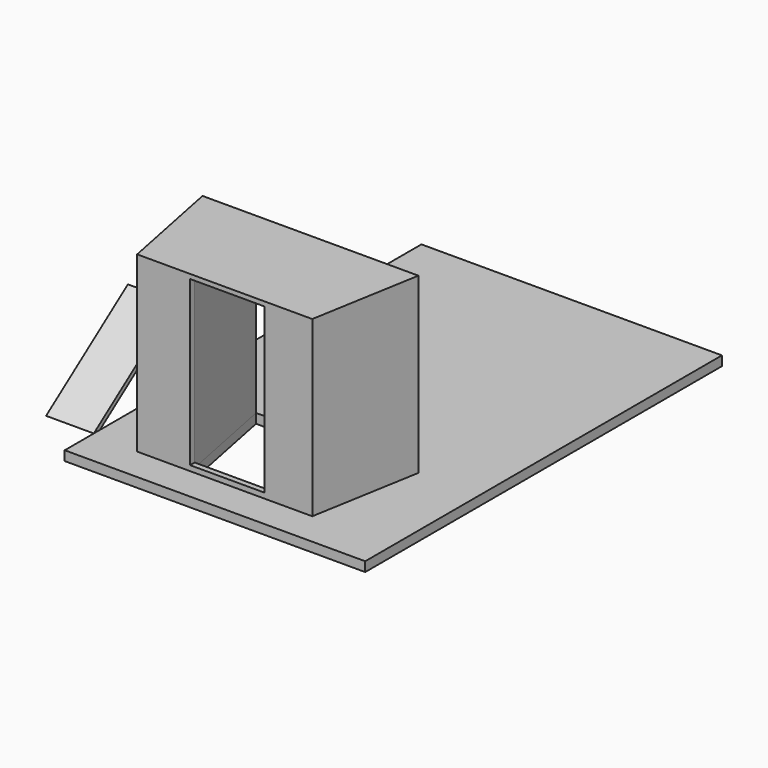
from build123d import *

# Parameters (mm, degrees)
F0_W        = 157.48
F0_H        = 233.68
F1_DEPTH    = 5
F3_DEPTH    = 91
F6_T        = 3
F6_T3_DEPTH = 64.2794708824
F6_T5_DEPTH = 72.7802281678
F6_T7_DEPTH = 63.9911646968
F4_W        = 61.3570176065
F4_H        = 85.9
F7_DEPTH    = 71
F8_DEPTH    = 27.4
F3_FACE1_W  = 58.2794708824
F3_FACE1_H  = 91
F3_FACE2_W  = 57.9911646968
F3_FACE2_H  = 91
F10_DEPTH   = 25


# Not quite as in the source:
# - a shell that OpenCascade refuses in one call is made with other operations: the cavity is built on its own and cut out


with BuildPart() as f1:
    # F0 (on Top) → F1 (new body)
    with BuildSketch(Plane.XY):
        with Locations((-51.8874652431, -0.1439023763)):
            Rectangle(F0_W, F0_H)
    extrude(amount=F1_DEPTH)

    # F2 (on face) → F3 (join)
    with BuildSketch(Plane.XY.offset(5)):
        Polygon((-93.2051390409, -42.2472283244), (-81.7390158772, -99.3876233697), (-14.9587877095, -99.3876233697), (-5.0617964007, -42.2472283244), align=None)
    extrude(amount=F3_DEPTH)

    # F6: shell of thickness 3, made by hand


with BuildPart() as f6_core1:
    # F6_t2: copy of F1
    add(f1.part)

    # the walls: a layer under each face that stays
    f6_faces = [f6_core1.faces().sort_by_distance(p)[0] for p in [
        (-51.8874652431, 116.6960976237, 2.5),
        (26.8525347569, -0.1439023763, 2.5),
        (-130.6274652431, -0.1439023763, 2.5),
        (-51.8874652431, -0.1439023763, 0),
        (-51.8874652431, -0.1439023763, 5),
        (-51.8874652431, -116.9839023763, 2.5),
        (-87.4720774591, -70.8174258471, 50.5),
        (-48.3489017934, -99.3876233697, 50.5),
        (-10.0102920551, -70.8174258471, 50.5),
        (-49.1334677208, -70.8174258471, 96),
    ]]
    thicken(f6_faces, amount=-F6_T, mode=Mode.SUBTRACT)

    # F6_s4 → F6_t3 (cut)
    with BuildSketch(Plane(origin=(3.9513966172, -19.6914301777, 0), x_dir=(0, 0, 1), z_dir=(0.196743776, -0.9804549386, 0))):
        Polygon((5.03, 99.7253181003), (2, 99.6953181003), (2, 96.6953181003), (5, 96.6953181003), align=None)
    extrude(amount=F6_T3_DEPTH, mode=Mode.SUBTRACT)

    # F6_s6 → F6_t5 (cut)
    with BuildSketch(Plane.YZ.offset(-84.7390158772)):
        Polygon((-99.4176233697, 5.03), (-99.3876233697, 2), (-96.3876233697, 2), (-96.3876233697, 5), align=None)
    extrude(amount=F6_T5_DEPTH, mode=Mode.SUBTRACT)

    # F6_s8 → F6_t7 (cut)
    with BuildSketch(Plane(origin=(-17.6607081625, -101.9643050803, 0), x_dir=(0, 0, 1), z_dir=(0.1706637789, 0.9853293229, 0))):
        Polygon((5.03, 2.2525352128), (2, 2.2225352128), (2, -0.7774647872), (5, -0.7774647872), align=None)
    extrude(amount=F6_T7_DEPTH, mode=Mode.SUBTRACT)


with BuildPart() as f1_1:
    add(f1.part)

    # what is left inside the walls is the cavity
    f6_cavity = [f6_core1.part.solids().sort_by_distance(p)[0] for p in [
        (-62.799045, -42.277228, 48),
    ]]
    add(f6_cavity, mode=Mode.SUBTRACT)

    # F4 (on face) → F7 (cut)
    with BuildSketch(Plane.XZ.offset(99.3876233697)):
        with Locations((-48.3198929578, 50.7050797723)):
            Rectangle(F4_W, F4_H)
    extrude(amount=-F7_DEPTH, mode=Mode.SUBTRACT)

    # F8 (cut): a face of the model
    f8_faces = [f1_1.faces().sort_by_distance(p)[0] for p in [
        (-48.771647492, -68.0475987274, 3),
    ]]
    extrude(f8_faces, amount=-F8_DEPTH, mode=Mode.SUBTRACT)

    # F9 (on face) + F3_face1 (on face) + F8_face (on face) + F8_face1 (on face) + F3_face2 (on face) → F10 (join)
    with BuildSketch(Plane(origin=(-130.6274652431, 0, 0), x_dir=(0, -1, 0), z_dir=(-1, 0, 0))):
        Polygon((93.9320304401, 5), (97.9320304401, 5), (44.34663196, 43.8861806393), (43.1026443839, 41.8861806393), align=None)
    with BuildSketch(Plane(origin=(-87.4720774591, -70.8174258471, 50.5), x_dir=(0.196743776, -0.9804549386, 0), z_dir=(-0.9804549386, -0.196743776, 0))):
        Rectangle(F3_FACE1_W, F3_FACE1_H)
    with BuildSketch(Plane(origin=(-84.7132721029, -69.3174258471, 46.5), x_dir=(-0.196743776, 0.9804549386, 0), z_dir=(0.9804549386, 0.196743776, 0))):
        Polygon((-27.6098334121, 46.5), (-27.6098334121, -46.5), (27.6098334121, -46.5), (27.6098334121, -41.5), (27.6098334121, 46.5), align=None)
    with BuildSketch(Plane(origin=(-12.7951521703, -69.3174258471, 46.5), x_dir=(-0.1706637789, -0.9853293229, 0), z_dir=(-0.9853293229, 0.1706637789, 0))):
        Polygon((-27.4732486828, -41.5), (-27.4732486828, -46.5), (27.4732486828, -46.5), (27.4732486828, 46.5), (-27.4732486828, 46.5), align=None)
    with BuildSketch(Plane(origin=(-10.0102920551, -70.8174258471, 50.5), x_dir=(0.1706637789, 0.9853293229, 0), z_dir=(0.9853293229, -0.1706637789, 0))):
        Rectangle(F3_FACE2_W, F3_FACE2_H)
    extrude(amount=F10_DEPTH, dir=(-1, 0, 0))


solid = f1_1.part
